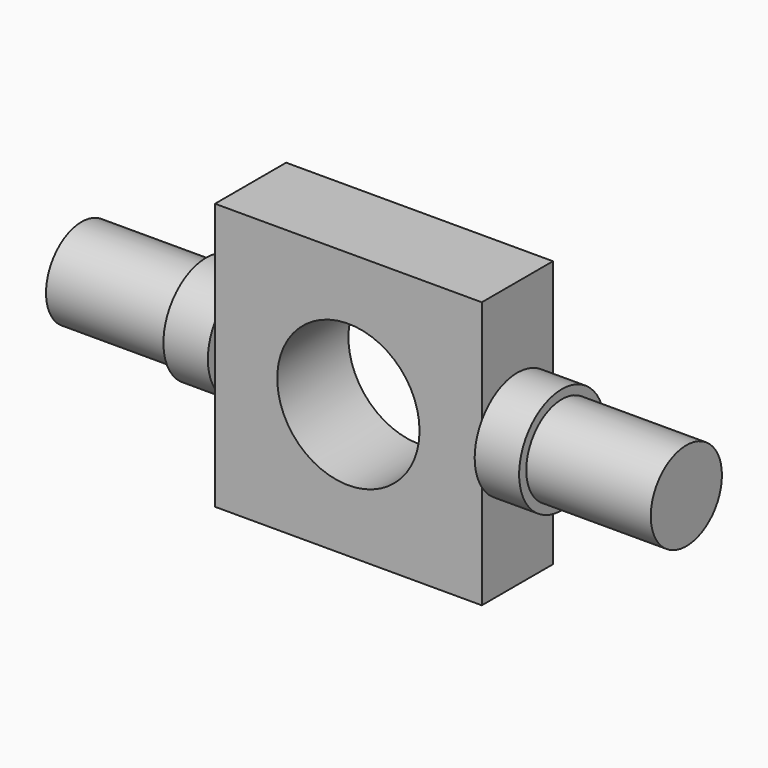
from build123d import *

# Parameters (mm, degrees)
F0_W      = 15
F0_H      = 15
F1_DEPTH  = 5
F2_R      = 4
F3_DEPTH  = 25
F4_R      = 3
F5_DEPTH  = 2.5
F10_R     = 2.5
F11_DEPTH = 7


with BuildPart() as f1:
    # F0 (on Front) → F1 (new body)
    with BuildSketch(Plane.XZ):
        with Locations((-2.477283068, 5.5355651764)):
            Rectangle(F0_W, F0_H)
    extrude(amount=F1_DEPTH)

    # F2 (on face) → F3 (cut)
    with BuildSketch(Plane.XZ.offset(5)):
        with Locations((-2.477283068, 5.5355651764)):
            Circle(F2_R)
    extrude(amount=-F3_DEPTH, mode=Mode.SUBTRACT)

    # F4 (on face) → F5 (join)
    with BuildSketch(Plane.YZ.offset(5.022716932)):
        with Locations((-2.5, 5.5355651764)):
            Circle(F4_R)
    extrude(amount=F5_DEPTH)

    # F10 (on face) → F11 (join)
    with BuildSketch(Plane.YZ.offset(7.522716932)):
        with Locations((-2.5, 5.5355651764)):
            Circle(F10_R)
    extrude(amount=F11_DEPTH)

    # F12: F1 across plane


with BuildPart() as f1_1:
    add(f1.part)
    add(f1.part.mirror(Plane(origin=(-2.477283068, 0, 13.0355651764), x_dir=(0, -1, 0), z_dir=(-1, 0, 0))))


solid = f1_1.part
